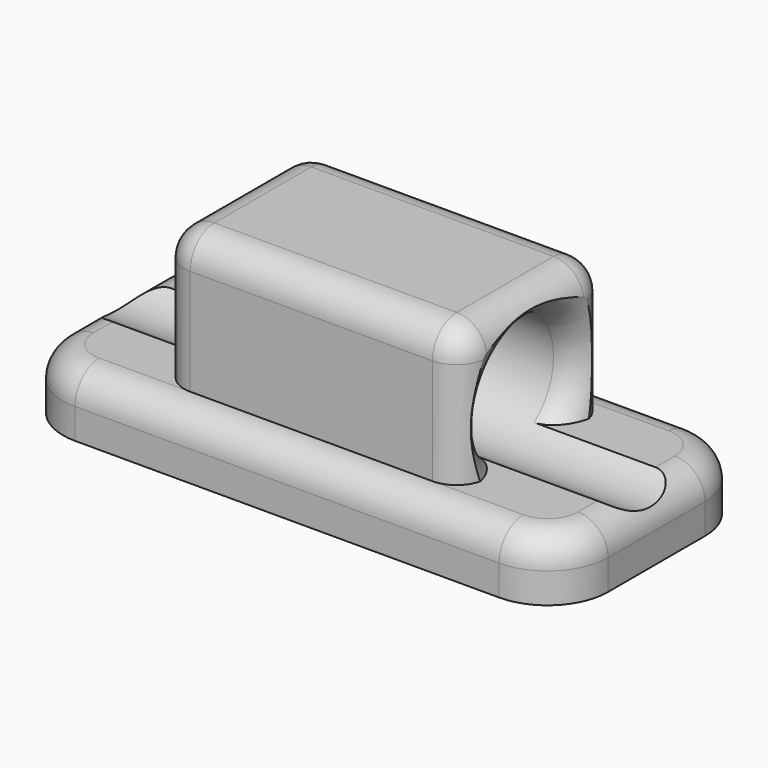
from build123d import *

# Parameters (mm, degrees)
F0_W         = 5
F0_H         = 3
F1_DEPTH     = 3.25
F0_W_2       = 9
F0_H_2       = 4
F2_DEPTH     = 1
F5_DEPTH     = 12.5
F6_T1_DEPTH  = 4
F6_T3_DEPTH  = 2
F6_T5_DEPTH  = 1.75
F6_S9_W      = 0.5
F6_S9_H      = 0.5
F6_T10_DEPTH = 0.5
F6_S15_W     = 0.5
F6_S15_H     = 0.5
F6_T16_DEPTH = 0.5
F6_S21_W     = 0.5
F6_S21_H     = 0.5
F6_T22_DEPTH = 0.5
F6_S27_W     = 0.5
F6_S27_H     = 0.5
F6_T28_DEPTH = 0.5
F6_T34_ANGLE = 359.64
F7_T1_DEPTH  = 15
F7_T3_DEPTH  = 7.4
F7_T5_DEPTH  = 7.4
F8_T1_DEPTH  = 3.5
F8_T4_ANGLE  = 90
F8_T6_ANGLE  = 90
F8_T8_ANGLE  = 90
F8_T10_ANGLE = 90


# Not quite as in the source:
# - a fillet or chamfer that OpenCascade refuses, or shapes differently, is made with other operations: its cross-section is extruded or revolved along the edge and cut away or added
# - a feature names something its author has since deleted; it is built from what else it names


with BuildPart() as f1:
    # F0 (on Top) → F1 (new body)
    with BuildSketch(Plane.XY):
        with Locations((4.5, 2)):
            Rectangle(F0_W, F0_H)
    extrude(amount=F1_DEPTH)

    # F0 (on Top) → F2 (join)
    with BuildSketch(Plane.XY):
        with Locations((4.5, 2)):
            Rectangle(F0_W_2, F0_H_2)
        with Locations((4.5, 2)):
            Rectangle(F0_W, F0_H, mode=Mode.SUBTRACT)
    extrude(amount=F2_DEPTH)

    # F4 (on face) → F5 (cut, symmetric)
    with BuildSketch(Plane.YZ.offset(7)):
        with BuildLine():
            Line((2.6, 1), (1.4, 1))
            ThreePointArc((1.4, 1), (2, 0.8), (2.6, 1))
        make_face()
        with BuildLine():
            ThreePointArc((2.6, 1), (2.894427191, 1.3527864045), (3, 1.8))
            ThreePointArc((3, 1.8), (1.5527864045, 2.694427191), (1.4, 1))
            Line((1.4, 1), (2.6, 1))
        make_face()
    extrude(amount=F5_DEPTH, both=True, mode=Mode.SUBTRACT)

    # F6: fillet of radius 0.5 on 9 edges, made by hand

    # F6_s2 → F6_t1 (cut)
    with BuildSketch(Plane.YZ.offset(2.5)):
        with BuildLine():
            ThreePointArc((0.5, 2.75), (0.6464466094, 3.1035533906), (1, 3.25))
            Line((1, 3.25), (0.5, 3.25))
            Line((0.5, 3.25), (0.5, 2.75))
        make_face()
        with BuildLine():
            ThreePointArc((3, 3.25), (3.3535533906, 3.1035533906), (3.5, 2.75))
            Line((3.5, 2.75), (3.5, 3.25))
            Line((3.5, 3.25), (3, 3.25))
        make_face()
    extrude(amount=F6_T1_DEPTH, mode=Mode.SUBTRACT)

    # F6_s4 → F6_t3 (cut)
    with BuildSketch(Plane.XZ.offset(-3)):
        with BuildLine():
            ThreePointArc((6.5, 3.25), (6.8535533906, 3.1035533906), (7, 2.75))
            Line((7, 2.75), (7, 3.25))
            Line((7, 3.25), (6.5, 3.25))
        make_face()
        with BuildLine():
            ThreePointArc((2, 2.75), (2.1464466094, 3.1035533906), (2.5, 3.25))
            Line((2.5, 3.25), (2, 3.25))
            Line((2, 3.25), (2, 2.75))
        make_face()
    extrude(amount=F6_T3_DEPTH, mode=Mode.SUBTRACT)

    # F6_s6 → F6_t5 (cut)
    with BuildSketch(Plane.XY.offset(1)):
        with BuildLine():
            ThreePointArc((6.5, 0.5), (6.8535533906, 0.6464466094), (7, 1))
            Line((7, 1), (7, 0.5))
            Line((7, 0.5), (6.5, 0.5))
        make_face()
        with BuildLine():
            ThreePointArc((6.5, 3.5), (6.8535533906, 3.3535533906), (7, 3))
            Line((7, 3), (7, 3.5))
            Line((7, 3.5), (6.5, 3.5))
        make_face()
        with BuildLine():
            ThreePointArc((2, 1), (2.1464466094, 0.6464466094), (2.5, 0.5))
            Line((2.5, 0.5), (2, 0.5))
            Line((2, 0.5), (2, 1))
        make_face()
        with BuildLine():
            ThreePointArc((2, 3), (2.1464466094, 3.3535533906), (2.5, 3.5))
            Line((2.5, 3.5), (2, 3.5))
            Line((2, 3.5), (2, 3))
        make_face()
    extrude(amount=F6_T5_DEPTH, mode=Mode.SUBTRACT)


with BuildPart() as f6_tool8:
    # F6_s9 → F6_t10 (new body)
    with BuildSketch(Plane.YZ.offset(2.5)):
        with Locations((0.75, 3)):
            Rectangle(F6_S9_W, F6_S9_H)
    extrude(amount=-F6_T10_DEPTH)

    # F6_s11 → F6_t12 (revolve, cut)
    with BuildSketch(Plane(origin=(2.5, 1, 2.75), x_dir=(0, 0.7071067812, -0.7071067812), z_dir=(0, 0.7071067812, 0.7071067812))):
        with BuildLine():
            ThreePointArc((0, -0.5), (0.5, 0), (0, 0.5))
            Line((0, 0.5), (0, -0.5))
        make_face()
    revolve(axis=Axis((2.5, 1, 2.75), (-1, 0, 0)), mode=Mode.SUBTRACT)


with BuildPart() as f1_1:
    add(f1.part)

    # F6_t7: cut F6_tool8
    add(f6_tool8.part, mode=Mode.SUBTRACT)


with BuildPart() as f6_tool14:
    # F6_s15 → F6_t16 (new body)
    with BuildSketch(Plane.YZ.offset(6.5)):
        with Locations((0.75, 3)):
            Rectangle(F6_S15_W, F6_S15_H)
    extrude(amount=F6_T16_DEPTH)

    # F6_s17 → F6_t18 (revolve, cut)
    with BuildSketch(Plane(origin=(6.5, 1, 2.75), x_dir=(0, 0.7071067812, -0.7071067812), z_dir=(0, -0.7071067812, -0.7071067812))):
        with BuildLine():
            ThreePointArc((0, -0.5), (0.5, 0), (0, 0.5))
            Line((0, 0.5), (0, -0.5))
        make_face()
    revolve(axis=Axis((6.5, 1, 2.75), (1, 0, 0)), mode=Mode.SUBTRACT)


with BuildPart() as f1_2:
    add(f1_1.part)

    # F6_t13: cut F6_tool14
    add(f6_tool14.part, mode=Mode.SUBTRACT)


with BuildPart() as f6_tool20:
    # F6_s21 → F6_t22 (new body)
    with BuildSketch(Plane.YZ.offset(6.5)):
        with Locations((3.25, 3)):
            Rectangle(F6_S21_W, F6_S21_H)
    extrude(amount=F6_T22_DEPTH)

    # F6_s23 → F6_t24 (revolve, cut)
    with BuildSketch(Plane(origin=(6.5, 3, 2.75), x_dir=(0, -0.7071067812, -0.7071067812), z_dir=(0, -0.7071067812, 0.7071067812))):
        with BuildLine():
            ThreePointArc((0, -0.5), (0.5, 0), (0, 0.5))
            Line((0, 0.5), (0, -0.5))
        make_face()
    revolve(axis=Axis((6.5, 3, 2.75), (1, 0, 0)), mode=Mode.SUBTRACT)


with BuildPart() as f1_3:
    add(f1_2.part)

    # F6_t19: cut F6_tool20
    add(f6_tool20.part, mode=Mode.SUBTRACT)


with BuildPart() as f6_tool26:
    # F6_s27 → F6_t28 (new body)
    with BuildSketch(Plane.YZ.offset(2.5)):
        with Locations((3.25, 3)):
            Rectangle(F6_S27_W, F6_S27_H)
    extrude(amount=-F6_T28_DEPTH)

    # F6_s29 → F6_t30 (revolve, cut)
    with BuildSketch(Plane(origin=(2.5, 3, 2.75), x_dir=(0, -0.7071067812, -0.7071067812), z_dir=(0, 0.7071067812, -0.7071067812))):
        with BuildLine():
            ThreePointArc((0, -0.5), (0.5, 0), (0, 0.5))
            Line((0, 0.5), (0, -0.5))
        make_face()
    revolve(axis=Axis((2.5, 3, 2.75), (-1, 0, 0)), mode=Mode.SUBTRACT)


with BuildPart() as f1_4:
    add(f1_3.part)

    # F6_t25: cut F6_tool26
    add(f6_tool26.part, mode=Mode.SUBTRACT)


with BuildPart() as f6_tool32:
    # F6_s33 → F6_t34 (revolve)
    with BuildSketch(Plane(origin=(0, 2.0056350904, 0.0063009092), x_dir=(1, 0, 0), z_dir=(0, -0.9999950652, -0.0031415875))):
        with BuildLine():
            ThreePointArc((6.5, 0.7937079424), (6.8535533906, 0.647261333), (7, 0.2937079424))
            Line((7, 0.2937079424), (7, 0.7937079424))
            Line((7, 0.7937079424), (6.5, 0.7937079424))
        make_face()
    revolve(axis=Axis((7, 2, 1.8), (1, 0, 0)), revolution_arc=F6_T34_ANGLE)

    split(bisect_by=Plane.XY.offset(1), keep=Keep.TOP)


with BuildPart() as f1_5:
    add(f1_4.part)

    # F6_t31: cut F6_tool32
    add(f6_tool32.part, mode=Mode.SUBTRACT)

    # F7: fillet of radius 0.5 on 4 edges, made by hand

    # F7_s2 → F7_t1 (cut)
    with BuildSketch(Plane.YZ.offset(-3)):
        with BuildLine():
            ThreePointArc((3.5, 1), (3.8535533906, 0.8535533906), (4, 0.5))
            Line((4, 0.5), (4.01, 0.5))
            Line((4.01, 0.5), (4.01, 1.01))
            Line((4.01, 1.01), (3.5, 1.01))
            Line((3.5, 1.01), (3.5, 1))
        make_face()
        with BuildLine():
            ThreePointArc((0.5, 1), (0.1464466094, 0.8535533906), (0, 0.5))
            Line((0, 0.5), (-0.01, 0.5))
            Line((-0.01, 0.5), (-0.01, 1.01))
            Line((-0.01, 1.01), (0.5, 1.01))
            Line((0.5, 1.01), (0.5, 1))
        make_face()
    extrude(amount=F7_T1_DEPTH, mode=Mode.SUBTRACT)

    # F7_s4 → F7_t3 (cut)
    with BuildSketch(Plane.XZ.offset(-4.4)):
        with BuildLine():
            ThreePointArc((0.5, 1), (0.1464466094, 0.8535533906), (0, 0.5))
            Line((0, 0.5), (-0.01, 0.5))
            Line((-0.01, 0.5), (-0.01, 1.01))
            Line((-0.01, 1.01), (0.5, 1.01))
            Line((0.5, 1.01), (0.5, 1))
        make_face()
    extrude(amount=F7_T3_DEPTH, mode=Mode.SUBTRACT)

    # F7_s6 → F7_t5 (cut)
    with BuildSketch(Plane.XZ.offset(-7)):
        with BuildLine():
            ThreePointArc((8.5, 1), (8.8535533906, 0.8535533906), (9, 0.5))
            Line((9, 0.5), (9.01, 0.5))
            Line((9.01, 0.5), (9.01, 1.01))
            Line((9.01, 1.01), (8.5, 1.01))
            Line((8.5, 1.01), (8.5, 1))
        make_face()
    extrude(amount=F7_T5_DEPTH, mode=Mode.SUBTRACT)

    # F8: fillet of radius 1 on 4 edges, made by hand

    # F8_s2 → F8_t1 (cut)
    with BuildSketch(Plane.XY.offset(-2.5)):
        with BuildLine():
            ThreePointArc((9, 1), (8.7071067812, 0.2928932188), (8, 0))
            Line((8, 0), (9, 0))
            Line((9, 0), (9, 1))
        make_face()
        with BuildLine():
            ThreePointArc((9, 3), (8.7071067812, 3.7071067812), (8, 4))
            Line((8, 4), (9, 4))
            Line((9, 4), (9, 3))
        make_face()
        with BuildLine():
            ThreePointArc((0, 1), (0.2928932188, 0.2928932188), (1, 0))
            Line((1, 0), (0, 0))
            Line((0, 0), (0, 1))
        make_face()
        with BuildLine():
            ThreePointArc((0, 3), (0.2928932188, 3.7071067812), (1, 4))
            Line((1, 4), (0, 4))
            Line((0, 4), (0, 3))
        make_face()
    extrude(amount=F8_T1_DEPTH, mode=Mode.SUBTRACT)

    # F8_s3 → F8_t4 (revolve, cut)
    with BuildSketch(Plane.YZ.offset(1)):
        with BuildLine():
            ThreePointArc((3.5, 1), (3.8535533906, 0.8535533906), (4, 0.5))
            Line((4, 0.5), (4, 1))
            Line((4, 1), (3.5, 1))
        make_face()
    revolve(axis=Axis((1, 3, 1), (0, 0, 1)), revolution_arc=F8_T4_ANGLE, mode=Mode.SUBTRACT)

    # F8_s5 → F8_t6 (revolve, cut)
    with BuildSketch(Plane.XZ.offset(-1)):
        with BuildLine():
            ThreePointArc((0.5, 1), (0.1464466094, 0.8535533906), (0, 0.5))
            Line((0, 0.5), (0, 1))
            Line((0, 1), (0.5, 1))
        make_face()
    revolve(axis=Axis((1, 1, 1), (0, 0, 1)), revolution_arc=F8_T6_ANGLE, mode=Mode.SUBTRACT)

    # F8_s7 → F8_t8 (revolve, cut)
    with BuildSketch(Plane.XZ.offset(-3)):
        with BuildLine():
            ThreePointArc((8.5, 1), (8.8535533906, 0.8535533906), (9, 0.5))
            Line((9, 0.5), (9, 1))
            Line((9, 1), (8.5, 1))
        make_face()
    revolve(axis=Axis((8, 3, 1), (0, 0, 1)), revolution_arc=F8_T8_ANGLE, mode=Mode.SUBTRACT)

    # F8_s9 → F8_t10 (revolve, cut)
    with BuildSketch(Plane.YZ.offset(8)):
        with BuildLine():
            ThreePointArc((0.5, 1), (0.1464466094, 0.8535533906), (0, 0.5))
            Line((0, 0.5), (0, 1))
            Line((0, 1), (0.5, 1))
        make_face()
    revolve(axis=Axis((8, 1, 1), (0, 0, 1)), revolution_arc=F8_T10_ANGLE, mode=Mode.SUBTRACT)


solid = f1_5.part
